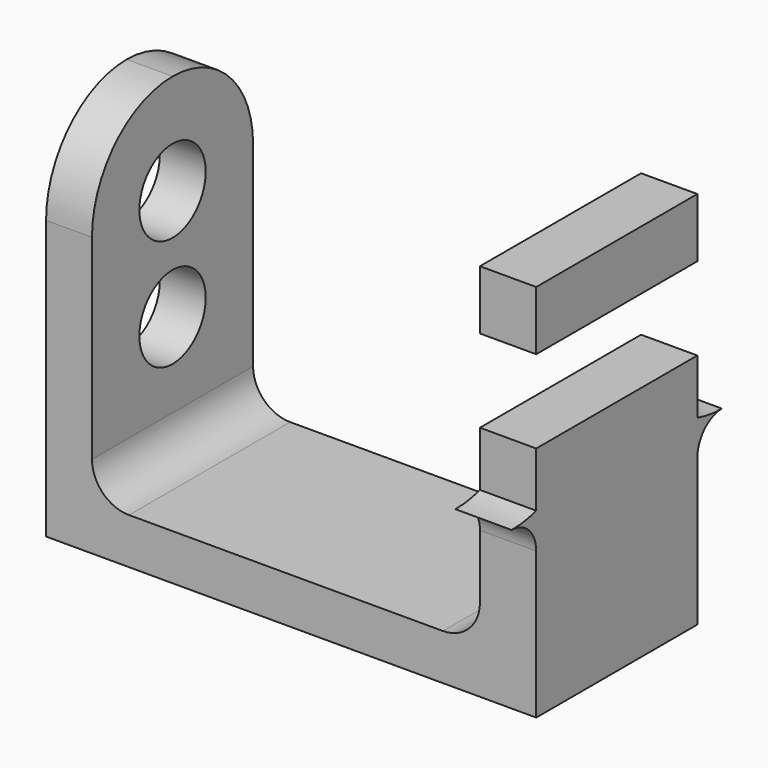
from build123d import *

# Parameters (mm, degrees)
F1_DEPTH = 17.272
F2_R     = 7.112
F3_DEPTH = 7.874
F5_DEPTH = 9.652
F4_W     = 34.544
F4_H     = 14.224
F6_DEPTH = 9.652


# Not quite as in the source:
# - a feature names something its author has since deleted; it is built from what else it names


with BuildPart() as f1:
    # F0 (on Front) → F1 (new body, symmetric)
    with BuildSketch(Plane.XZ):
        with BuildLine():
            ThreePointArc((14.224, 7.874), (9.7338719395, 9.7338719395), (7.874, 14.224))
            Line((7.874, 14.224), (7.874, 7.874))
            Line((7.874, 7.874), (14.224, 7.874))
        make_face()
        with BuildLine():
            Line((74.422, 7.874), (74.422, 14.224))
            ThreePointArc((74.422, 14.224), (72.5621280605, 9.7338719395), (68.072, 7.874))
            Line((68.072, 7.874), (74.422, 7.874))
        make_face()
        Polygon((0, 65.024), (0, 0), (84.074, 0), (84.074, 65.024), (74.422, 65.024), (74.422, 14.224), (74.422, 7.874), (68.072, 7.874), (14.224, 7.874), (7.874, 7.874), (7.874, 14.224), (7.874, 65.024), align=None)
    extrude(amount=F1_DEPTH, both=True)

    # F2 (on face) → F3 (cut, through all)
    with BuildSketch(Plane(origin=(0, 0, 0), x_dir=(0, -1, 0), z_dir=(-1, 0, 0))):
        with BuildLine():
            ThreePointArc((-17.272, 47.752), (-12.2131483247, 59.9651483247), (0, 65.024))
            Line((0, 65.024), (-17.272, 65.024))
            Line((-17.272, 65.024), (-17.272, 47.752))
        make_face()
        with BuildLine():
            ThreePointArc((0, 65.024), (12.2131483247, 59.9651483247), (17.272, 47.752))
            Line((17.272, 47.752), (17.272, 65.024))
            Line((17.272, 65.024), (0, 65.024))
        make_face()
        with Locations((0, 47.752)):
            Circle(F2_R)
        with Locations((0, 28.702)):
            Circle(F2_R)
    extrude(amount=-F3_DEPTH, mode=Mode.SUBTRACT)

    # F4 (on face) → F5 (join, through all)
    with BuildSketch(Plane.YZ.offset(84.074)):
        with BuildLine():
            Line((-17.272, 25.5601424724), (-17.272, 31.2439539618))
            ThreePointArc((-17.272, 31.2439539618), (-19.8794356336, 30.6578954767), (-22.5460674157, 30.4810903008))
            ThreePointArc((-22.5460674157, 30.4810903008), (-18.8131622494, 28.8978853564), (-17.272, 25.1474270113))
            Line((-17.272, 25.1474270113), (-17.272, 25.5601424724))
        make_face()
        with BuildLine():
            ThreePointArc((22.5460674157, 30.4810903008), (19.8794356336, 30.6578954767), (17.272, 31.2439539618))
            Line((17.272, 31.2439539618), (17.272, 30.48))
            Line((17.272, 30.48), (17.272, 25.1474270113))
            ThreePointArc((17.272, 25.1474270113), (18.8131622494, 28.8978853564), (22.5460674157, 30.4810903008))
        make_face()
    extrude(amount=-F5_DEPTH)

    # F4 (on face) → F6 (cut, through all)
    with BuildSketch(Plane.YZ.offset(84.074)):
        with Locations((0, 47.752)):
            Rectangle(F4_W, F4_H)
    extrude(amount=-F6_DEPTH, mode=Mode.SUBTRACT)


solid = f1.part
